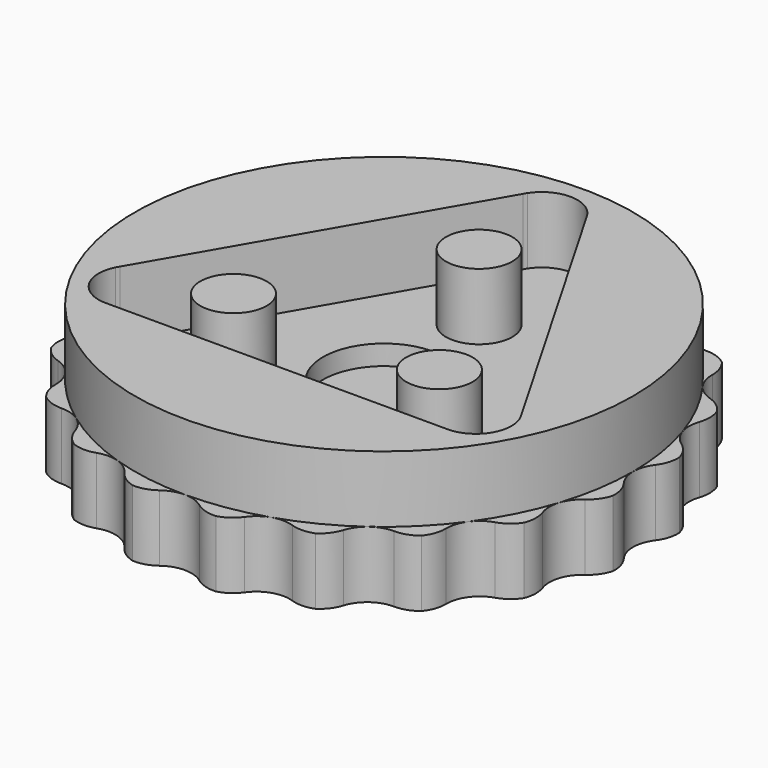
from build123d import *

# Parameters (mm, degrees)
F1_DEPTH     = 10
F2_R         = 37.5
F3_DEPTH     = 10
F5_DEPTH     = 10
F6_R         = 5
F7_DEPTH     = 10
F8_R         = 9.1971929399
F9_DEPTH     = 3
F10_T1_DEPTH = 23.3255587161


# Not quite as in the source:
# - a fillet or chamfer that OpenCascade refuses, or shapes differently, is made with other operations: its cross-section is extruded or revolved along the edge and cut away or added


with BuildPart() as f1:
    # F0 (on Top) → F1 (new body)
    with BuildSketch(Plane.XY):
        with BuildLine():
            ThreePointArc((-8.3027897066, 39.1288088636), (-11.5881372891, 35.6646193611), (-16.2822388164, 36.5361286828))
            ThreePointArc((-16.2822388164, 36.5361286828), (-18.1596199896, 35.6402609675), (-19.9878891624, 34.6480055246))
            ThreePointArc((-19.9878891624, 34.6480055246), (-22.041946961, 30.3381372891), (-26.7756139979, 29.7164347632))
            ThreePointArc((-26.7756139979, 29.7164347632), (-28.2842712475, 28.2842712475), (-29.7164347632, 26.7756139979))
            ThreePointArc((-29.7164347632, 26.7756139979), (-30.3381372891, 22.041946961), (-34.6480055246, 19.9878891624))
            ThreePointArc((-34.6480055246, 19.9878891624), (-35.6402609675, 18.1596199896), (-36.5361286828, 16.2822388164))
            ThreePointArc((-36.5361286828, 16.2822388164), (-35.6646193611, 11.5881372891), (-39.1288088636, 8.3027897066))
            ThreePointArc((-39.1288088636, 8.3027897066), (-39.5075336238, 6.2573786016), (-39.7794117647, 4.1950446546))
            ThreePointArc((-39.7794117647, 4.1950446546), (-37.5, 0), (-39.7794117647, -4.1950446546))
            ThreePointArc((-39.7794117647, -4.1950446546), (-39.5075336238, -6.2573786016), (-39.1288088636, -8.3027897066))
            ThreePointArc((-39.1288088636, -8.3027897066), (-35.6646193611, -11.5881372891), (-36.5361286828, -16.2822388164))
            ThreePointArc((-36.5361286828, -16.2822388164), (-35.6402609675, -18.1596199896), (-34.6480055246, -19.9878891624))
            ThreePointArc((-34.6480055246, -19.9878891624), (-30.3381372891, -22.041946961), (-29.7164347632, -26.7756139979))
            ThreePointArc((-29.7164347632, -26.7756139979), (-28.2842712475, -28.2842712475), (-26.7756139979, -29.7164347632))
            ThreePointArc((-26.7756139979, -29.7164347632), (-22.041946961, -30.3381372891), (-19.9878891624, -34.6480055246))
            ThreePointArc((-19.9878891624, -34.6480055246), (-18.1596199896, -35.6402609675), (-16.2822388164, -36.5361286828))
            ThreePointArc((-16.2822388164, -36.5361286828), (-11.5881372891, -35.6646193611), (-8.3027897066, -39.1288088636))
            ThreePointArc((-8.3027897066, -39.1288088636), (-6.2573786016, -39.5075336238), (-4.1950446546, -39.7794117647))
            ThreePointArc((-4.1950446546, -39.7794117647), (0, -37.5), (4.1950446546, -39.7794117647))
            ThreePointArc((4.1950446546, -39.7794117647), (6.2573786016, -39.5075336238), (8.3027897066, -39.1288088636))
            ThreePointArc((8.3027897066, -39.1288088636), (11.5881372891, -35.6646193611), (16.2822388164, -36.5361286828))
            ThreePointArc((16.2822388164, -36.5361286828), (18.1596199896, -35.6402609675), (19.9878891624, -34.6480055246))
            ThreePointArc((19.9878891624, -34.6480055246), (22.041946961, -30.3381372891), (26.7756139979, -29.7164347632))
            ThreePointArc((26.7756139979, -29.7164347632), (28.2842712475, -28.2842712475), (29.7164347632, -26.7756139979))
            ThreePointArc((29.7164347632, -26.7756139979), (30.3381372891, -22.041946961), (34.6480055246, -19.9878891624))
            ThreePointArc((34.6480055246, -19.9878891624), (35.6402609675, -18.1596199896), (36.5361286828, -16.2822388164))
            ThreePointArc((36.5361286828, -16.2822388164), (35.6646193611, -11.5881372891), (39.1288088636, -8.3027897066))
            ThreePointArc((39.1288088636, -8.3027897066), (39.5075336238, -6.2573786016), (39.7794117647, -4.1950446546))
            ThreePointArc((39.7794117647, -4.1950446546), (37.5, 0), (39.7794117647, 4.1950446546))
            ThreePointArc((39.7794117647, 4.1950446546), (39.5075336238, 6.2573786016), (39.1288088636, 8.3027897066))
            ThreePointArc((39.1288088636, 8.3027897066), (35.6646193611, 11.5881372891), (36.5361286828, 16.2822388164))
            ThreePointArc((36.5361286828, 16.2822388164), (35.6402609675, 18.1596199896), (34.6480055246, 19.9878891624))
            ThreePointArc((34.6480055246, 19.9878891624), (30.3381372891, 22.041946961), (29.7164347632, 26.7756139979))
            ThreePointArc((29.7164347632, 26.7756139979), (28.2842712475, 28.2842712475), (26.7756139979, 29.7164347632))
            ThreePointArc((26.7756139979, 29.7164347632), (22.041946961, 30.3381372891), (19.9878891624, 34.6480055246))
            ThreePointArc((19.9878891624, 34.6480055246), (18.1596199896, 35.6402609675), (16.2822388164, 36.5361286828))
            ThreePointArc((16.2822388164, 36.5361286828), (11.5881372891, 35.6646193611), (8.3027897066, 39.1288088636))
            ThreePointArc((8.3027897066, 39.1288088636), (6.2573786016, 39.5075336238), (4.1950446546, 39.7794117647))
            ThreePointArc((4.1950446546, 39.7794117647), (0, 37.5), (-4.1950446546, 39.7794117647))
            ThreePointArc((-4.1950446546, 39.7794117647), (-6.2573786016, 39.5075336238), (-8.3027897066, 39.1288088636))
        make_face()
    extrude(amount=F1_DEPTH)

    # F2 (on face) → F3 (join)
    with BuildSketch(Plane.XY.offset(10)):
        Circle(F2_R)
    extrude(amount=F3_DEPTH)

    # F4 (on face) → F5 (cut)
    with BuildSketch(Plane.XY.offset(20)):
        with BuildLine():
            ThreePointArc((4.7728963756, 32.1476198215), (4.6469213614, 32.3787263275), (4.5097647633, 32.6033771431))
            Line((4.5097647633, 32.6033771431), (4.7728963756, 32.1476198215))
        make_face()
        with BuildLine():
            Line((4.7728963756, 32.1476198215), (4.5097647633, 32.6033771431))
            ThreePointArc((4.5097647633, 32.6033771431), (0, 35.0616276264), (-4.5097647633, 32.6033771431))
            Line((-4.5097647633, 32.6033771431), (-4.7728963756, 32.1476198215))
            Line((-4.7728963756, 32.1476198215), (-30.2271036244, -11.9403603999))
            Line((-30.2271036244, -11.9403603999), (-30.4902352367, -12.3961177214))
            ThreePointArc((-30.4902352367, -12.3961177214), (-30.3642602225, -17.5308138132), (-25.9804704734, -20.2072594216))
            Line((-25.9804704734, -20.2072594216), (-25.4542072488, -20.2072594216))
            Line((-25.4542072488, -20.2072594216), (25.4542072488, -20.2072594216))
            Line((25.4542072488, -20.2072594216), (25.9804704734, -20.2072594216))
            ThreePointArc((25.9804704734, -20.2072594216), (30.3642602225, -17.5308138132), (30.4902352367, -12.3961177214))
            Line((30.4902352367, -12.3961177214), (30.2271036244, -11.9403603999))
            Line((30.2271036244, -11.9403603999), (4.7728963756, 32.1476198215))
        make_face()
        with BuildLine():
            Line((-4.7728963756, 32.1476198215), (-4.5097647633, 32.6033771431))
            ThreePointArc((-4.5097647633, 32.6033771431), (-4.6469213614, 32.3787263275), (-4.7728963756, 32.1476198215))
        make_face()
        with BuildLine():
            ThreePointArc((30.4902352367, -12.3961177214), (30.3642602225, -12.1650112154), (30.2271036244, -11.9403603999))
            Line((30.2271036244, -11.9403603999), (30.4902352367, -12.3961177214))
        make_face()
        with BuildLine():
            Line((-30.4902352367, -12.3961177214), (-30.2271036244, -11.9403603999))
            ThreePointArc((-30.2271036244, -11.9403603999), (-30.3642602225, -12.1650112154), (-30.4902352367, -12.3961177214))
        make_face()
        with BuildLine():
            ThreePointArc((25.4542072488, -20.2072594216), (25.7173388611, -20.2137151121), (25.9804704734, -20.2072594216))
            Line((25.9804704734, -20.2072594216), (25.4542072488, -20.2072594216))
        make_face()
        with BuildLine():
            Line((-25.4542072488, -20.2072594216), (-25.9804704734, -20.2072594216))
            ThreePointArc((-25.9804704734, -20.2072594216), (-25.7173388611, -20.2137151121), (-25.4542072488, -20.2072594216))
        make_face()
    extrude(amount=-F5_DEPTH, mode=Mode.SUBTRACT)

    # F6 (on face) → F7 (join)
    with BuildSketch(Plane.XY.offset(10)):
        with Locations((0, 17.8978583449)):
            Circle(F6_R)
        with Locations((-15.5, -8.9489291724)):
            Circle(F6_R)
        with Locations((15.5, -8.9489291724)):
            Circle(F6_R)
    extrude(amount=F7_DEPTH)

    # F8 (on face) → F9 (cut)
    with BuildSketch(Plane.XY.offset(10)):
        Circle(F8_R)
    extrude(amount=-F9_DEPTH, mode=Mode.SUBTRACT)

    # F10: fillet of radius 5 on 40 edges, made by hand

    # F10_s2 → F10_t1 (cut)
    with BuildSketch(Plane.XY.offset(-6.662779358)):
        with BuildLine():
            ThreePointArc((-6.8346764933, -39.4117647059), (-4.8177398507, -39.3482516952), (-2.9901709658, -38.4926470588))
            ThreePointArc((-2.9901709658, -38.4926470588), (-3.649763243, -39.0825114089), (-4.1950446546, -39.7794117647))
            ThreePointArc((-4.1950446546, -39.7794117647), (-5.517923363, -39.6175784439), (-6.8346764933, -39.4117647059))
        make_face()
        with BuildLine():
            ThreePointArc((-9.0510605178, -37.5326964593), (-7.5773355939, -38.9111746679), (-5.6787414567, -39.5948468297))
            ThreePointArc((-5.6787414567, -39.5948468297), (-6.9946480443, -39.3836882318), (-8.3027897066, -39.1288088636))
            ThreePointArc((-8.3027897066, -39.1288088636), (-8.606029093, -38.2975160162), (-9.0510605178, -37.5326964593))
        make_face()
        with BuildLine():
            ThreePointArc((2.9901709658, -38.4926470588), (4.8177398507, -39.3482516952), (6.8346764933, -39.4117647059))
            ThreePointArc((6.8346764933, -39.4117647059), (5.517923363, -39.6175784439), (4.1950446546, -39.7794117647))
            ThreePointArc((4.1950446546, -39.7794117647), (3.649763243, -39.0825114089), (2.9901709658, -38.4926470588))
        make_face()
        with BuildLine():
            ThreePointArc((5.6787414567, -39.5948468297), (7.5773355939, -38.9111746679), (9.0510605178, -37.5326964593))
            ThreePointArc((9.0510605178, -37.5326964593), (8.606029093, -38.2975160162), (8.3027897066, -39.1288088636))
            ThreePointArc((8.3027897066, -39.1288088636), (6.9946480443, -39.3836882318), (5.6787414567, -39.5948468297))
        make_face()
        with BuildLine():
            ThreePointArc((14.7387036815, -35.6846691702), (16.7412213516, -35.9336476912), (18.6790686882, -35.3707844547))
            ThreePointArc((18.6790686882, -35.3707844547), (17.490361986, -35.9734240461), (16.2822388164, -36.5361286828))
            ThreePointArc((16.2822388164, -36.5361286828), (15.5482913234, -36.0418382811), (14.7387036815, -35.6846691702))
        make_face()
        with BuildLine():
            ThreePointArc((17.6362846268, -35.9021094723), (19.2306886363, -34.665200754), (20.2063111354, -32.8987840246))
            ThreePointArc((20.2063111354, -32.8987840246), (20.0194033397, -33.7636929213), (19.9878891624, -34.6480055246))
            ThreePointArc((19.9878891624, -34.6480055246), (18.8225345665, -35.2946482132), (17.6362846268, -35.9021094723))
        make_face()
        with BuildLine():
            ThreePointArc((25.0445093903, -29.3836272335), (27.0259554636, -29.0016078868), (28.6950234951, -27.8674653784))
            ThreePointArc((28.6950234951, -27.8674653784), (27.7507221152, -28.8079402611), (26.7756139979, -29.7164347632))
            ThreePointArc((26.7756139979, -29.7164347632), (25.9248443178, -29.4731389041), (25.0445093903, -29.3836272335))
        make_face()
        with BuildLine():
            ThreePointArc((27.8674653784, -28.6950234951), (29.0016078868, -27.0259554636), (29.3836272335, -25.0445093903))
            ThreePointArc((29.3836272335, -25.0445093903), (29.4731389041, -25.9248443178), (29.7164347632, -26.7756139979))
            ThreePointArc((29.7164347632, -26.7756139979), (28.8079402611, -27.7507221152), (27.8674653784, -28.6950234951))
        make_face()
        with BuildLine():
            ThreePointArc((32.8987840246, -20.2063111354), (34.665200754, -19.2306886363), (35.9021094723, -17.6362846268))
            ThreePointArc((35.9021094723, -17.6362846268), (35.2946482132, -18.8225345665), (34.6480055246, -19.9878891624))
            ThreePointArc((34.6480055246, -19.9878891624), (33.7636929213, -20.0194033397), (32.8987840246, -20.2063111354))
        make_face()
        with BuildLine():
            ThreePointArc((35.3707844547, -18.6790686882), (35.9336476912, -16.7412213516), (35.6846691702, -14.7387036815))
            ThreePointArc((35.6846691702, -14.7387036815), (36.0418382811, -15.5482913234), (36.5361286828, -16.2822388164))
            ThreePointArc((36.5361286828, -16.2822388164), (35.9734240461, -17.490361986), (35.3707844547, -18.6790686882))
        make_face()
        with BuildLine():
            ThreePointArc((37.5326964593, -9.0510605178), (38.9111746679, -7.5773355939), (39.5948468297, -5.6787414567))
            ThreePointArc((39.5948468297, -5.6787414567), (39.3836882318, -6.9946480443), (39.1288088636, -8.3027897066))
            ThreePointArc((39.1288088636, -8.3027897066), (38.2975160162, -8.606029093), (37.5326964593, -9.0510605178))
        make_face()
        with BuildLine():
            ThreePointArc((39.4117647059, -6.8346764933), (39.3482516952, -4.8177398507), (38.4926470588, -2.9901709658))
            ThreePointArc((38.4926470588, -2.9901709658), (39.0825114089, -3.649763243), (39.7794117647, -4.1950446546))
            ThreePointArc((39.7794117647, -4.1950446546), (39.6175784439, -5.517923363), (39.4117647059, -6.8346764933))
        make_face()
        with BuildLine():
            ThreePointArc((38.4926470588, 2.9901709658), (39.3482516952, 4.8177398507), (39.4117647059, 6.8346764933))
            ThreePointArc((39.4117647059, 6.8346764933), (39.6175784439, 5.517923363), (39.7794117647, 4.1950446546))
            ThreePointArc((39.7794117647, 4.1950446546), (39.0825114089, 3.649763243), (38.4926470588, 2.9901709658))
        make_face()
        with BuildLine():
            ThreePointArc((39.5948468297, 5.6787414567), (38.9111746679, 7.5773355939), (37.5326964593, 9.0510605178))
            ThreePointArc((37.5326964593, 9.0510605178), (38.2975160162, 8.606029093), (39.1288088636, 8.3027897066))
            ThreePointArc((39.1288088636, 8.3027897066), (39.3836882318, 6.9946480443), (39.5948468297, 5.6787414567))
        make_face()
        with BuildLine():
            ThreePointArc((35.6846691702, 14.7387036815), (35.9336476912, 16.7412213516), (35.3707844547, 18.6790686882))
            ThreePointArc((35.3707844547, 18.6790686882), (35.9734240461, 17.490361986), (36.5361286828, 16.2822388164))
            ThreePointArc((36.5361286828, 16.2822388164), (36.0418382811, 15.5482913234), (35.6846691702, 14.7387036815))
        make_face()
        with BuildLine():
            ThreePointArc((29.3836272335, 25.0445093903), (29.0016078868, 27.0259554636), (27.8674653784, 28.6950234951))
            ThreePointArc((27.8674653784, 28.6950234951), (28.8079402611, 27.7507221152), (29.7164347632, 26.7756139979))
            ThreePointArc((29.7164347632, 26.7756139979), (29.4731389041, 25.9248443178), (29.3836272335, 25.0445093903))
        make_face()
        with BuildLine():
            ThreePointArc((28.6950234951, 27.8674653784), (27.0259554636, 29.0016078868), (25.0445093903, 29.3836272335))
            ThreePointArc((25.0445093903, 29.3836272335), (25.9248443178, 29.4731389041), (26.7756139979, 29.7164347632))
            ThreePointArc((26.7756139979, 29.7164347632), (27.7507221152, 28.8079402611), (28.6950234951, 27.8674653784))
        make_face()
        with BuildLine():
            ThreePointArc((35.9021094723, 17.6362846268), (34.665200754, 19.2306886363), (32.8987840246, 20.2063111354))
            ThreePointArc((32.8987840246, 20.2063111354), (33.7636929213, 20.0194033397), (34.6480055246, 19.9878891624))
            ThreePointArc((34.6480055246, 19.9878891624), (35.2946482132, 18.8225345665), (35.9021094723, 17.6362846268))
        make_face()
        with BuildLine():
            ThreePointArc((20.2063111354, 32.8987840246), (19.2306886363, 34.665200754), (17.6362846268, 35.9021094723))
            ThreePointArc((17.6362846268, 35.9021094723), (18.8225345665, 35.2946482132), (19.9878891624, 34.6480055246))
            ThreePointArc((19.9878891624, 34.6480055246), (20.0194033397, 33.7636929213), (20.2063111354, 32.8987840246))
        make_face()
        with BuildLine():
            ThreePointArc((14.7387036815, 35.6846691702), (16.7412213516, 35.9336476912), (18.6790686882, 35.3707844547))
            ThreePointArc((18.6790686882, 35.3707844547), (17.490361986, 35.9734240461), (16.2822388164, 36.5361286828))
            ThreePointArc((16.2822388164, 36.5361286828), (15.5482913234, 36.0418382811), (14.7387036815, 35.6846691702))
        make_face()
        with BuildLine():
            ThreePointArc((2.9901709658, 38.4926470588), (4.8177398507, 39.3482516952), (6.8346764933, 39.4117647059))
            ThreePointArc((6.8346764933, 39.4117647059), (5.517923363, 39.6175784439), (4.1950446546, 39.7794117647))
            ThreePointArc((4.1950446546, 39.7794117647), (3.649763243, 39.0825114089), (2.9901709658, 38.4926470588))
        make_face()
        with BuildLine():
            ThreePointArc((5.6787414567, 39.5948468297), (7.5773355939, 38.9111746679), (9.0510605178, 37.5326964593))
            ThreePointArc((9.0510605178, 37.5326964593), (8.606029093, 38.2975160162), (8.3027897066, 39.1288088636))
            ThreePointArc((8.3027897066, 39.1288088636), (6.9946480443, 39.3836882318), (5.6787414567, 39.5948468297))
        make_face()
        with BuildLine():
            ThreePointArc((-18.6790686882, -35.3707844547), (-16.7412213516, -35.9336476912), (-14.7387036815, -35.6846691702))
            ThreePointArc((-14.7387036815, -35.6846691702), (-15.5482913234, -36.0418382811), (-16.2822388164, -36.5361286828))
            ThreePointArc((-16.2822388164, -36.5361286828), (-17.490361986, -35.9734240461), (-18.6790686882, -35.3707844547))
        make_face()
        with BuildLine():
            ThreePointArc((-20.2063111354, -32.8987840246), (-19.2306886363, -34.665200754), (-17.6362846268, -35.9021094723))
            ThreePointArc((-17.6362846268, -35.9021094723), (-18.8225345665, -35.2946482132), (-19.9878891624, -34.6480055246))
            ThreePointArc((-19.9878891624, -34.6480055246), (-20.0194033397, -33.7636929213), (-20.2063111354, -32.8987840246))
        make_face()
        with BuildLine():
            ThreePointArc((-28.6950234951, -27.8674653784), (-27.0259554636, -29.0016078868), (-25.0445093903, -29.3836272335))
            ThreePointArc((-25.0445093903, -29.3836272335), (-25.9248443178, -29.4731389041), (-26.7756139979, -29.7164347632))
            ThreePointArc((-26.7756139979, -29.7164347632), (-27.7507221152, -28.8079402611), (-28.6950234951, -27.8674653784))
        make_face()
        with BuildLine():
            ThreePointArc((-29.3836272335, -25.0445093903), (-29.0016078868, -27.0259554636), (-27.8674653784, -28.6950234951))
            ThreePointArc((-27.8674653784, -28.6950234951), (-28.8079402611, -27.7507221152), (-29.7164347632, -26.7756139979))
            ThreePointArc((-29.7164347632, -26.7756139979), (-29.4731389041, -25.9248443178), (-29.3836272335, -25.0445093903))
        make_face()
        with BuildLine():
            ThreePointArc((-35.9021094723, -17.6362846268), (-34.665200754, -19.2306886363), (-32.8987840246, -20.2063111354))
            ThreePointArc((-32.8987840246, -20.2063111354), (-33.7636929213, -20.0194033397), (-34.6480055246, -19.9878891624))
            ThreePointArc((-34.6480055246, -19.9878891624), (-35.2946482132, -18.8225345665), (-35.9021094723, -17.6362846268))
        make_face()
        with BuildLine():
            ThreePointArc((-35.6846691702, -14.7387036815), (-35.9336476912, -16.7412213516), (-35.3707844547, -18.6790686882))
            ThreePointArc((-35.3707844547, -18.6790686882), (-35.9734240461, -17.490361986), (-36.5361286828, -16.2822388164))
            ThreePointArc((-36.5361286828, -16.2822388164), (-36.0418382811, -15.5482913234), (-35.6846691702, -14.7387036815))
        make_face()
        with BuildLine():
            ThreePointArc((-39.5948468297, -5.6787414567), (-38.9111746679, -7.5773355939), (-37.5326964593, -9.0510605178))
            ThreePointArc((-37.5326964593, -9.0510605178), (-38.2975160162, -8.606029093), (-39.1288088636, -8.3027897066))
            ThreePointArc((-39.1288088636, -8.3027897066), (-39.3836882318, -6.9946480443), (-39.5948468297, -5.6787414567))
        make_face()
        with BuildLine():
            ThreePointArc((-38.4926470588, -2.9901709658), (-39.3482516952, -4.8177398507), (-39.4117647059, -6.8346764933))
            ThreePointArc((-39.4117647059, -6.8346764933), (-39.6175784439, -5.517923363), (-39.7794117647, -4.1950446546))
            ThreePointArc((-39.7794117647, -4.1950446546), (-39.0825114089, -3.649763243), (-38.4926470588, -2.9901709658))
        make_face()
        with BuildLine():
            ThreePointArc((-39.4117647059, 6.8346764933), (-39.3482516952, 4.8177398507), (-38.4926470588, 2.9901709658))
            ThreePointArc((-38.4926470588, 2.9901709658), (-39.0825114089, 3.649763243), (-39.7794117647, 4.1950446546))
            ThreePointArc((-39.7794117647, 4.1950446546), (-39.6175784439, 5.517923363), (-39.4117647059, 6.8346764933))
        make_face()
        with BuildLine():
            ThreePointArc((-37.5326964593, 9.0510605178), (-38.9111746679, 7.5773355939), (-39.5948468297, 5.6787414567))
            ThreePointArc((-39.5948468297, 5.6787414567), (-39.3836882318, 6.9946480443), (-39.1288088636, 8.3027897066))
            ThreePointArc((-39.1288088636, 8.3027897066), (-38.2975160162, 8.606029093), (-37.5326964593, 9.0510605178))
        make_face()
        with BuildLine():
            ThreePointArc((-35.3707844547, 18.6790686882), (-35.9336476912, 16.7412213516), (-35.6846691702, 14.7387036815))
            ThreePointArc((-35.6846691702, 14.7387036815), (-36.0418382811, 15.5482913234), (-36.5361286828, 16.2822388164))
            ThreePointArc((-36.5361286828, 16.2822388164), (-35.9734240461, 17.490361986), (-35.3707844547, 18.6790686882))
        make_face()
        with BuildLine():
            ThreePointArc((-32.8987840246, 20.2063111354), (-34.665200754, 19.2306886363), (-35.9021094723, 17.6362846268))
            ThreePointArc((-35.9021094723, 17.6362846268), (-35.2946482132, 18.8225345665), (-34.6480055246, 19.9878891624))
            ThreePointArc((-34.6480055246, 19.9878891624), (-33.7636929213, 20.0194033397), (-32.8987840246, 20.2063111354))
        make_face()
        with BuildLine():
            ThreePointArc((-27.8674653784, 28.6950234951), (-29.0016078868, 27.0259554636), (-29.3836272335, 25.0445093903))
            ThreePointArc((-29.3836272335, 25.0445093903), (-29.4731389041, 25.9248443178), (-29.7164347632, 26.7756139979))
            ThreePointArc((-29.7164347632, 26.7756139979), (-28.8079402611, 27.7507221152), (-27.8674653784, 28.6950234951))
        make_face()
        with BuildLine():
            ThreePointArc((-25.0445093903, 29.3836272335), (-27.0259554636, 29.0016078868), (-28.6950234951, 27.8674653784))
            ThreePointArc((-28.6950234951, 27.8674653784), (-27.7507221152, 28.8079402611), (-26.7756139979, 29.7164347632))
            ThreePointArc((-26.7756139979, 29.7164347632), (-25.9248443178, 29.4731389041), (-25.0445093903, 29.3836272335))
        make_face()
        with BuildLine():
            ThreePointArc((-17.6362846268, 35.9021094723), (-19.2306886363, 34.665200754), (-20.2063111354, 32.8987840246))
            ThreePointArc((-20.2063111354, 32.8987840246), (-20.0194033397, 33.7636929213), (-19.9878891624, 34.6480055246))
            ThreePointArc((-19.9878891624, 34.6480055246), (-18.8225345665, 35.2946482132), (-17.6362846268, 35.9021094723))
        make_face()
        with BuildLine():
            ThreePointArc((-14.7387036815, 35.6846691702), (-16.7412213516, 35.9336476912), (-18.6790686882, 35.3707844547))
            ThreePointArc((-18.6790686882, 35.3707844547), (-17.490361986, 35.9734240461), (-16.2822388164, 36.5361286828))
            ThreePointArc((-16.2822388164, 36.5361286828), (-15.5482913234, 36.0418382811), (-14.7387036815, 35.6846691702))
        make_face()
        with BuildLine():
            ThreePointArc((-5.6787414567, 39.5948468297), (-7.5773355939, 38.9111746679), (-9.0510605178, 37.5326964593))
            ThreePointArc((-9.0510605178, 37.5326964593), (-8.606029093, 38.2975160162), (-8.3027897066, 39.1288088636))
            ThreePointArc((-8.3027897066, 39.1288088636), (-6.9946480443, 39.3836882318), (-5.6787414567, 39.5948468297))
        make_face()
        with BuildLine():
            ThreePointArc((-2.9901709658, 38.4926470588), (-4.8177398507, 39.3482516952), (-6.8346764933, 39.4117647059))
            ThreePointArc((-6.8346764933, 39.4117647059), (-5.517923363, 39.6175784439), (-4.1950446546, 39.7794117647))
            ThreePointArc((-4.1950446546, 39.7794117647), (-3.649763243, 39.0825114089), (-2.9901709658, 38.4926470588))
        make_face()
    extrude(amount=F10_T1_DEPTH, mode=Mode.SUBTRACT)


solid = f1.part
